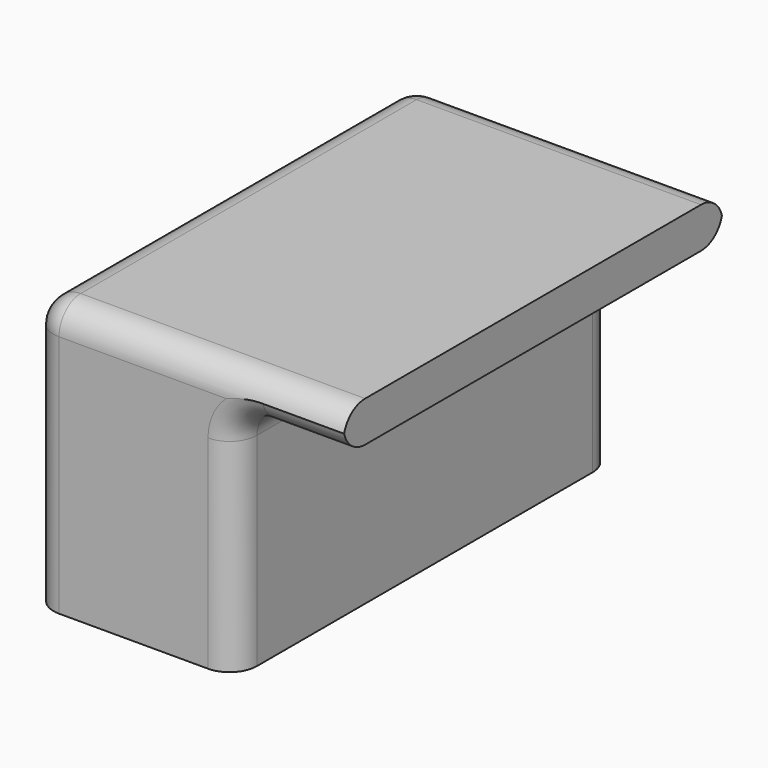
from build123d import *

# Parameters (mm, degrees)
F0_W         = 15
F0_H         = 35
F1_DEPTH     = 17
F2_W         = 23
F2_H         = 35
F3_DEPTH     = 3
F5_D         = 3
F5_DEPTH     = 10
F5_TIP       = 0.9012909285
F6_F1_R      = 2
F6_F2_R      = 2
F6_F3_R      = 2
F6_F4_R      = 2
F6_T5_DEPTH  = 20
F6_T7_DEPTH  = 11
F6_T10_ANGLE = 90
F6_T11_DEPTH = 20
F6_T13_DEPTH = 11
F6_T16_ANGLE = 90


# Not quite as in the source:
# - a fillet or chamfer that OpenCascade refuses, or shapes differently, is made with other operations: its cross-section is extruded or revolved along the edge and cut away or added


with BuildPart() as f1:
    # F0 (on Top) → F1 (new body)
    with BuildSketch(Plane.XY):
        Rectangle(F0_W, F0_H)
    extrude(amount=F1_DEPTH)

    # F2 (on face) → F3 (join)
    with BuildSketch(Plane.XY.offset(17)):
        with Locations((4, 0)):
            Rectangle(F2_W, F2_H)
    extrude(amount=F3_DEPTH)

    # F5
    with Locations(Plane(origin=(0, 0, 0), x_dir=(1, 0, 0), z_dir=(0, 0, -1))):
        with Locations((0, 9.5), (0, -9.5)):
            Hole(F5_D / 2, depth=F5_DEPTH)
            with Locations((0, 0, -(F5_DEPTH + F5_TIP / 2))):  # 118° drill point
                Cone(0, F5_D / 2, F5_TIP, mode=Mode.SUBTRACT)

    # F6: fillet of radius 2 on 8 edges, made by hand

    # F6_f1
    f6_f1_edges = [f1.edges().sort_by_distance(p)[0] for p in [
        (-7.5, 0, 20),
    ]]
    fillet(f6_f1_edges, radius=F6_F1_R)

    # F6_f2
    f6_f2_edges = [f1.edges().sort_by_distance(p)[0] for p in [
        (7.5, 0, 17),
    ]]
    fillet(f6_f2_edges, radius=F6_F2_R)

    # F6_f3
    f6_f3_edges = [f1.edges().sort_by_distance(p)[0] for p in [
        (5, -17.5, 20),
    ]]
    fillet(f6_f3_edges, radius=F6_F3_R)

    # F6_f4
    f6_f4_edges = [f1.edges().sort_by_distance(p)[0] for p in [
        (5, 17.5, 20),
    ]]
    fillet(f6_f4_edges, radius=F6_F4_R)

    # F6_s6 → F6_t5 (cut)
    with BuildSketch(Plane.XY.offset(-5)):
        with BuildLine():
            ThreePointArc((5.5, -17.5), (6.9142135624, -16.9142135624), (7.5, -15.5))
            Line((7.5, -15.5), (7.54, -15.5))
            Line((7.54, -15.5), (7.54, -17.54))
            Line((7.54, -17.54), (5.5, -17.54))
            Line((5.5, -17.54), (5.5, -17.5))
        make_face()
    extrude(amount=F6_T5_DEPTH, mode=Mode.SUBTRACT)

    # F6_s8 → F6_t7 (cut)
    with BuildSketch(Plane.YZ.offset(9.5)):
        with BuildLine():
            ThreePointArc((-17.5, 19), (-16.9142135624, 17.5857864376), (-15.5, 17))
            Line((-15.5, 17), (-15.5, 16.96))
            Line((-15.5, 16.96), (-17.54, 16.96))
            Line((-17.54, 16.96), (-17.54, 19))
            Line((-17.54, 19), (-17.5, 19))
        make_face()
    extrude(amount=F6_T7_DEPTH, mode=Mode.SUBTRACT)

    # F6_s9 → F6_t10 (revolve, cut)
    with BuildSketch(Plane.XY.offset(15)):
        with BuildLine():
            ThreePointArc((5.5, -17.5), (6.9142135624, -16.9142135624), (7.5, -15.5))
            Line((7.5, -15.5), (7.54, -15.5))
            Line((7.54, -15.5), (7.54, -17.54))
            Line((7.54, -17.54), (5.5, -17.54))
            Line((5.5, -17.54), (5.5, -17.5))
        make_face()
    revolve(axis=Axis((9.5, -17.5, 15), (0, 1, 0)), revolution_arc=F6_T10_ANGLE, mode=Mode.SUBTRACT)

    # F6_s12 → F6_t11 (cut)
    with BuildSketch(Plane.XY.offset(-5)):
        with BuildLine():
            ThreePointArc((5.5, 17.5), (6.9142135624, 16.9142135624), (7.5, 15.5))
            Line((7.5, 15.5), (7.54, 15.5))
            Line((7.54, 15.5), (7.54, 17.54))
            Line((7.54, 17.54), (5.5, 17.54))
            Line((5.5, 17.54), (5.5, 17.5))
        make_face()
    extrude(amount=F6_T11_DEPTH, mode=Mode.SUBTRACT)

    # F6_s14 → F6_t13 (cut)
    with BuildSketch(Plane.YZ.offset(9.5)):
        with BuildLine():
            ThreePointArc((17.5, 19), (16.9142135624, 17.5857864376), (15.5, 17))
            Line((15.5, 17), (15.5, 16.96))
            Line((15.5, 16.96), (17.54, 16.96))
            Line((17.54, 16.96), (17.54, 19))
            Line((17.54, 19), (17.5, 19))
        make_face()
    extrude(amount=F6_T13_DEPTH, mode=Mode.SUBTRACT)

    # F6_s15 → F6_t16 (revolve, cut)
    with BuildSketch(Plane.XY.offset(15)):
        with BuildLine():
            ThreePointArc((5.5, 17.5), (6.9142135624, 16.9142135624), (7.5, 15.5))
            Line((7.5, 15.5), (7.54, 15.5))
            Line((7.54, 15.5), (7.54, 17.54))
            Line((7.54, 17.54), (5.5, 17.54))
            Line((5.5, 17.54), (5.5, 17.5))
        make_face()
    revolve(axis=Axis((9.5, 17.5, 15), (0, 1, 0)), revolution_arc=F6_T16_ANGLE, mode=Mode.SUBTRACT)


solid = f1.part
